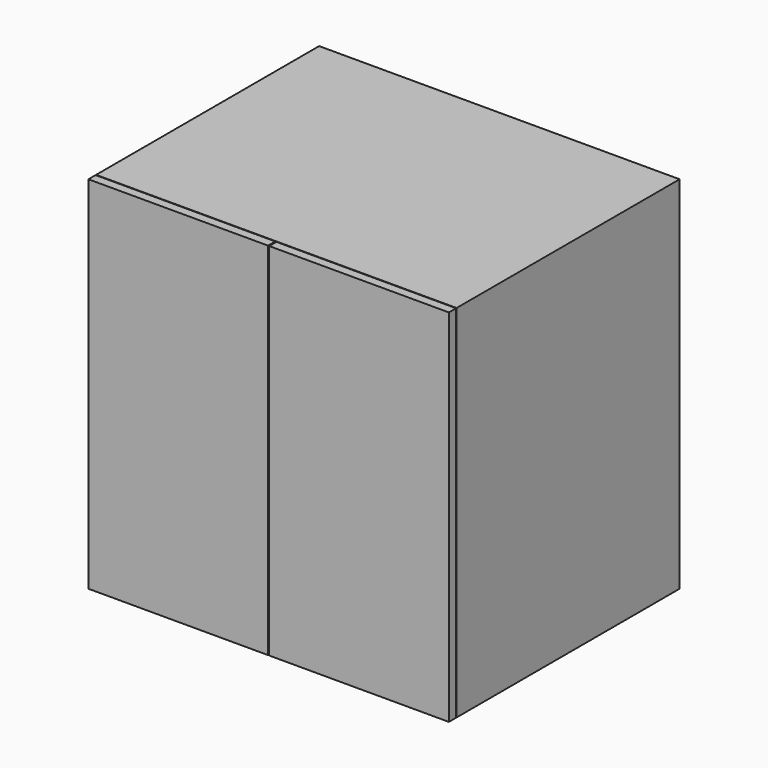
from build123d import *

# Parameters (mm, degrees)
F0_W     = 762
F0_H     = 589.28
F1_DEPTH = 762
F0_W_2   = 379.73
F0_H_2   = 19.05


# Not quite as in the source:
# - ends of sketch curves that miss each other by under 0.0002 mm in the source are joined


with BuildPart() as f1:
    # F0 (on Top) → F1 (new body)
    with BuildSketch(Plane.XY):
        with Locations((1.27, -0.635)):
            Rectangle(F0_W, F0_H)
    extrude(amount=F1_DEPTH)


with BuildPart() as f1b:
    # F0 (on Top) → F1, piece 2 (new body)
    with BuildSketch(Plane.XY):
        Polygon((382.27, -315.595), (382.27, -296.545), (2.54, -296.545), (2.54, -315.5950048161), align=None)
    extrude(amount=F1_DEPTH)


with BuildPart() as f1c:
    # F0 (on Top) → F1, piece 3 (new body)
    with BuildSketch(Plane.XY):
        with Locations((-189.865, -306.07)):
            Rectangle(F0_W_2, F0_H_2)
    extrude(amount=F1_DEPTH)


solid = Compound([f1.part, f1b.part, f1c.part])
